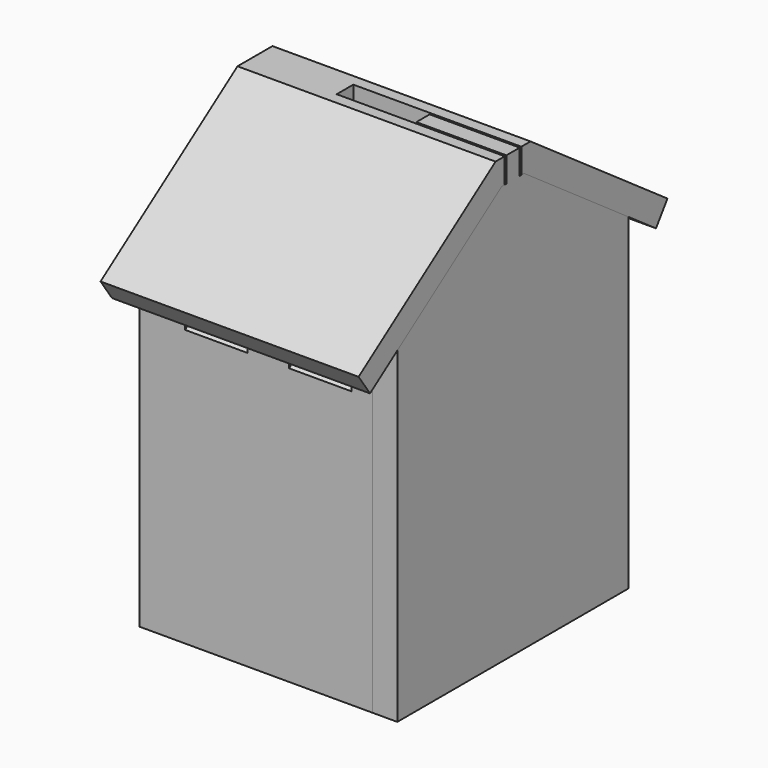
from build123d import *

# Parameters (mm, degrees)
F1_DEPTH       = 2.35
F3_W           = 8.5
F3_H           = 16.25
F4_DEPTH       = 1.5
F6_DEPTH       = 5
F7_W           = 3
F7_H           = 2
F8_REACH       = 22.1084224651
F13_R          = 1.25
F14_DEPTH      = 2.301
F16_DEPTH      = 1.2
F18_DEPTH      = 1.2
F20_DEPTH      = 6.875
F20_DEPTH_BACK = 1.2
F22_DEPTH      = 10
F24_DEPTH      = 1.2
F25_W          = 0.8
F25_H          = 1.2
F26_DEPTH      = 3.125
F27_W          = 8
F27_H          = 0.5
F28_DEPTH      = 15.7186173855
F30_DEPTH      = 10
F31_R          = 1.05
F32_DEPTH      = 1.2
F33_W          = 0.4
F33_H          = 14.25
F34_DEPTH      = 2
F35_W          = 0.4
F35_H          = 13.25
F36_DEPTH      = 2
F38_DEPTH      = 0.8


# Not quite as in the source:
# - a pattern or mirror of a feature is missing from the dataset's text; its kind, count and spacing are read off the source's solid


with BuildPart() as f1:
    # F0 (on Top) → F1 (new body, symmetric)
    with BuildSketch(Plane.XY):
        with BuildLine():
            Line((2.325, -1.225), (2.325, 0))
            ThreePointArc((2.325, 0), (0, 2.325), (-2.325, 0))
            Line((-2.325, 0), (-2.325, -1.225))
            Line((-2.325, -1.225), (2.325, -1.225))
        make_face()
    extrude(amount=F1_DEPTH, both=True)

    # F3 (on face) → F4 (join)
    with BuildSketch(Plane.XZ.offset(1.225)):
        with Locations((0, 4.075)):
            Rectangle(F3_W, F3_H)
    extrude(amount=F4_DEPTH)


with BuildPart() as f6:
    # F5 (on Right) → F6 (new body, symmetric)
    with BuildSketch(Plane.YZ):
        Polygon((-0.925, 15.9559049361), (-3.025, 15.9559049361), (-11.2515958122, 10.1955805346), (-10.5633040886, 9.2125980814), (-8.925, 10.3597509541), (-8.925, -5.35), (4.975, -5.35), (4.975, 10.3597509541), (6.6133040886, 9.2125980814), (7.3015958122, 10.1955805346), align=None)
        Polygon((-0.925, -4.15), (-3.025, -4.15), (-3.025, -3.05), (-7.725, -3.05), (-7.725, 11.2), (-3.025, 11.2), (-3.025, 12.3), (-0.925, 12.3), (-0.925, 11.2), (3.775, 11.2), (3.775, -3.05), (-0.925, -3.05), align=None, mode=Mode.SUBTRACT)
    extrude(amount=F6_DEPTH, both=True)

    f8_end = f6.faces().sort_by_distance((0, -5.375, 11.2))[0]
    # F7 (on face) → F8 (cut, up to a face of the model that its end follows)
    with BuildSketch(Plane(origin=(0, -2.7595782158, -1.932277469), x_dir=(1, 0, 0), z_dir=(0, -0.8191520443, -0.5735764364))):
        with Locations((-2.5, 12.6053808668)):
            Rectangle(F7_W, F7_H)
        with Locations((2.5, 12.6053808668)):
            Rectangle(F7_W, F7_H)
    f8_long = extrude(amount=-F8_REACH, mode=Mode.PRIVATE)
    f8 = split(f8_long, bisect_by=f8_end, keep=Keep.TOP, mode=Mode.PRIVATE)
    add(f8, mode=Mode.SUBTRACT)

    # F8_copies: F8 across plane
    add(f8.mirror(Plane.ZX.offset(-1.975)), mode=Mode.SUBTRACT)

    # F13 (on face) → F14 (cut, through all)
    with BuildSketch(Plane.XY.offset(-3.05)):
        with Locations((-3.125, 1.425)):
            Circle(F13_R)
        with Locations((0, 1.425)):
            Circle(F13_R)
        with Locations((3.125, 1.425)):
            Circle(F13_R)
    f14 = extrude(amount=-F14_DEPTH, mode=Mode.SUBTRACT)

    # F14_copies: F14 across plane
    add(f14.mirror(Plane(origin=(0, -1.975, 0), x_dir=(0, 0, -1), z_dir=(0, -1, 0))), mode=Mode.SUBTRACT)

    # F15 (on face) → F16 (join)
    with BuildSketch(Plane(origin=(-5, 0, 0), x_dir=(0, -1, 0), z_dir=(-1, 0, 0))):
        Polygon((3.025, 15.9559049361), (0.925, 15.9559049361), (-7.3015958122, 10.1955805346), (-6.6133040886, 9.2125980814), (-4.975, 10.3597509541), (-4.975, -5.35), (8.925, -5.35), (8.925, 10.3597509541), (10.5633040886, 9.2125980814), (11.2515958122, 10.1955805346), align=None)
    extrude(amount=F16_DEPTH)

    # F17 (on face) → F18 (join)
    with BuildSketch(Plane.YZ.offset(5)):
        Polygon((-0.925, 15.9559049361), (-3.025, 15.9559049361), (-11.2515958122, 10.1955805346), (-10.5633040886, 9.2125980814), (-2.6466414533, 14.7559049361), (-1.3033585467, 14.7559049361), (6.6133040886, 9.2125980814), (7.3015958122, 10.1955805346), align=None)
    extrude(amount=F18_DEPTH)

    # F19 (on face) → F20 (cut, two sides)
    with BuildSketch(Plane.YZ.offset(5)) as f20_sk:
        Polygon((-2.6466414533, 14.7559049361), (-4.7387776081, 13.2909754296), (-1.3033585467, 13.2909754296), (0.9687898419, 11.7), (0.9687898419, 11.2), (3.775, 11.2), (-1.3033585467, 14.7559049361), (-1.475, 14.7559049361), (-1.475, 15.9559049361), (-2.475, 15.9559049361), (-2.475, 14.7559049361), align=None)
    extrude(amount=-F20_DEPTH, mode=Mode.SUBTRACT)
    extrude(f20_sk.sketch, amount=F20_DEPTH_BACK, mode=Mode.SUBTRACT)

    # F21 (on face) → F22 (join, through all)
    with BuildSketch(Plane.YZ.offset(-5)):
        Polygon((3.775, 7.0485281374), (0.6235281374, 10.2), (-0.225, 9.3514718626), (3.775, 5.3514718626), align=None)
    extrude(amount=F22_DEPTH)

    # F27 (on face) → F28 (cut, through all)
    with BuildSketch(Plane(origin=(0, -4.7882359313, 4.7882359313), x_dir=(1, 0, 0), z_dir=(0, -0.7071067812, 0.7071067812))):
        with Locations((0, 7.9033901423)):
            Rectangle(F27_W, F27_H)
    extrude(amount=-F28_DEPTH, mode=Mode.SUBTRACT)

    # F29 (on face) → F30 (cut, through all)
    with BuildSketch(Plane.YZ.offset(5)):
        Polygon((-3.425, -3.05), (-7.325, -3.05), (-5.375, -4.15), align=None)
        Polygon((3.375, -3.05), (-0.525, -3.05), (1.425, -4.15), align=None)
    extrude(amount=-F30_DEPTH, mode=Mode.SUBTRACT)

    # F31 (on face) → F32 (cut, through all)
    with BuildSketch(Plane(origin=(0, 0, -5.35), x_dir=(1, 0, 0), z_dir=(0, 0, -1))):
        with Locations((0, 1.975)):
            Circle(F31_R)
    extrude(amount=-F32_DEPTH, mode=Mode.SUBTRACT)

    # F33 (on face) → F34 (join)
    with BuildSketch(Plane.YZ.offset(-5)):
        with Locations((-3.225, 4.075)):
            Rectangle(F33_W, F33_H)
        with Locations((-0.725, 4.075)):
            Rectangle(F33_W, F33_H)
    extrude(amount=F34_DEPTH)


with BuildPart() as f24:
    # F23 (on face) → F24 (new body, through all)
    with BuildSketch(Plane.YZ.offset(5)):
        Polygon((-2.6466414533, 14.7559049361), (-8.925, 10.3597509541), (-8.925, -5.35), (4.975, -5.35), (4.975, 10.3597509541), (-1.3033585467, 14.7559049361), (-1.575, 14.7559049361), (-1.575, 15.9559049361), (-2.375, 15.9559049361), (-2.375, 14.7559049361), align=None)
    extrude(amount=F24_DEPTH)

    # F25 (on face) → F26 (join, through all)
    with BuildSketch(Plane(origin=(5, 0, 0), x_dir=(0, -1, 0), z_dir=(-1, 0, 0))):
        with Locations((1.975, 15.3559049361)):
            Rectangle(F25_W, F25_H)
    extrude(amount=F26_DEPTH)

    # F35 (on face) → F36 (join)
    with BuildSketch(Plane(origin=(5, 0, 0), x_dir=(0, -1, 0), z_dir=(-1, 0, 0))):
        with Locations((3.225, 4.075)):
            Rectangle(F35_W, F35_H)
        with Locations((0.725, 4.075)):
            Rectangle(F35_W, F35_H)
    extrude(amount=F36_DEPTH)

    # F37 (on face) → F38 (join, through all)
    with BuildSketch(Plane(origin=(0, -1.575, 0), x_dir=(-1, 0, 0), z_dir=(0, 1, 0))):
        Polygon((-5, 13.5559049361), (-1.875, 14.7559049361), (-5, 14.7559049361), align=None)
    extrude(amount=-F38_DEPTH)


solid = Compound([f1.part, f6.part, f24.part])
